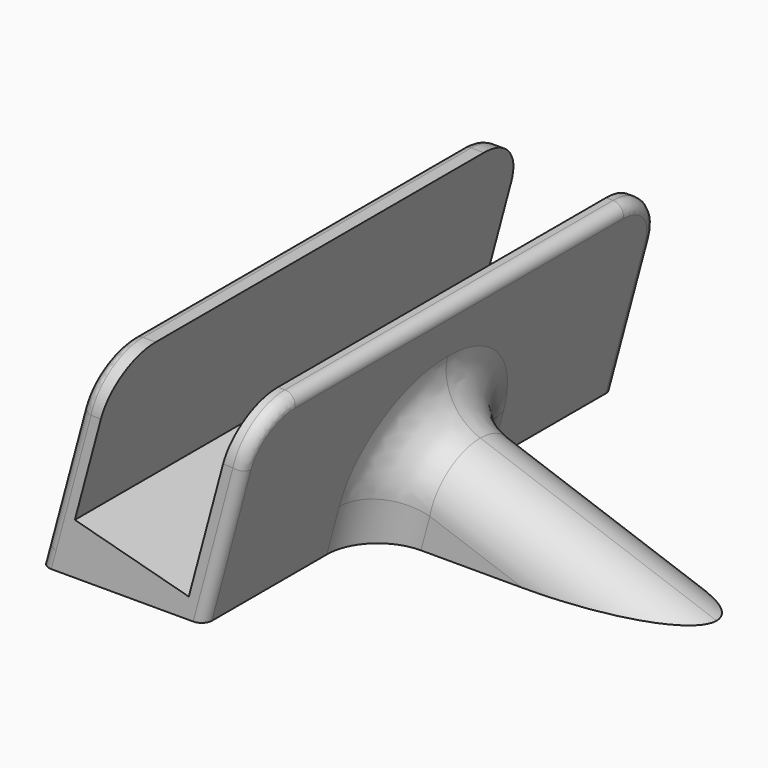
from build123d import *

# Parameters (mm, degrees)
F1_DEPTH = 25
F2_DEPTH = 5
F3_R     = 4.99999
F4_R     = 1


# Not quite as in the source:
# - a fillet or chamfer is up to 0.001 mm smaller than in the source, because OpenCascade refuses the exact size


with BuildPart() as f1:
    # F0 (on Front) → F1 (new body, symmetric)
    with BuildSketch(Plane.XZ):
        Polygon((4.6798147489, 17.465306413), (0, 0), (-11.1081470023, 2.9764190187), (-7.2258613258, 17.465306413), (-9.2258613258, 17.465306413), (-13.9056760747, 0), (-14.4415744596, -2), (1.4641016151, -2), (4.071958182, 7.7326532065), (6.6798147489, 17.465306413), align=None)
    extrude(amount=F1_DEPTH, both=True)

    # F0 (on Front) → F2 (join, symmetric)
    with BuildSketch(Plane.XZ):
        Polygon((31.4641016151, -2), (4.071958182, 7.7326532065), (1.4641016151, -2), align=None)
    extrude(amount=F2_DEPTH, both=True)

    # F3 (radius 5 in the source; OpenCascade refuses exactly that, so slightly less here)
    f3_edges = [f1.edges().sort_by_distance(p)[0] for p in [
        (2.76803, -5, 2.866327),
        (4.071958, 0, 7.732653),
        (2.76803, 5, 2.866327),
        (17.76803, 5, 2.866327),
        (17.76803, -5, 2.866327),
        (5.679815, -25, 17.465306),
        (-8.225861, -25, 17.465306),
        (-8.225861, 25, 17.465306),
        (5.679815, 25, 17.465306),
    ]]
    fillet(f3_edges, radius=F3_R)

    # F4
    f4_edges = [f1.edges().sort_by_distance(p)[0] for p in [
        (-9.225861, 0, 17.465306),
        (6.679815, 0, 17.465306),
    ]]
    fillet(f4_edges, radius=F4_R)


solid = f1.part
